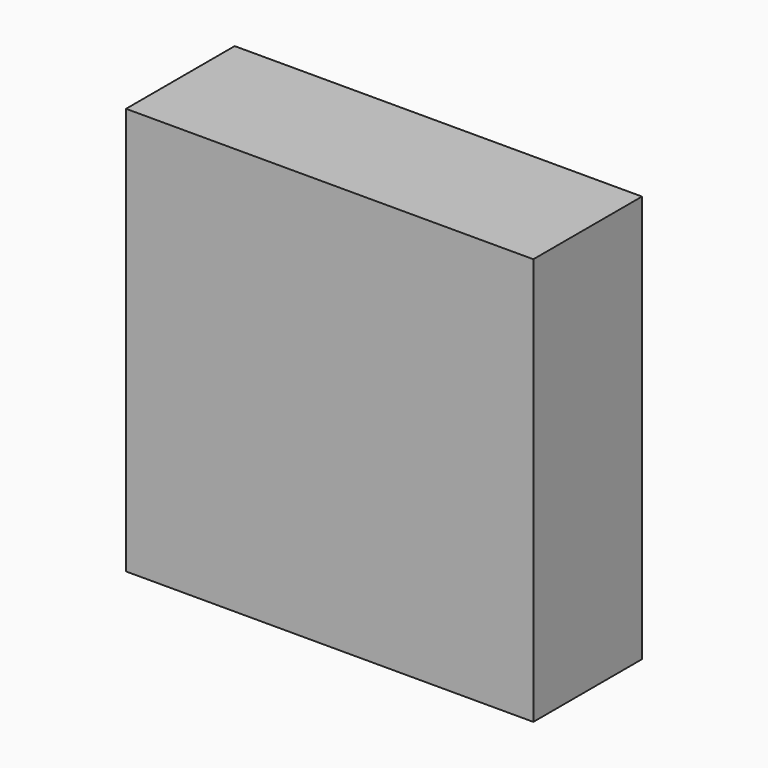
from build123d import *

# Parameters (mm, degrees)
F0_W     = 152.4
F0_H     = 152.4
F1_DEPTH = 50.8


# Not quite as in the source:
# - a feature names something its author has since deleted; it is built from what else it names


with BuildPart() as f1:
    # F0 (on Front) → F1 (new body)
    with BuildSketch(Plane.XZ):
        with Locations((1.3375543058, -9.8106506928)):
            Rectangle(F0_W, F0_H)
    extrude(amount=F1_DEPTH)


solid = f1.part
